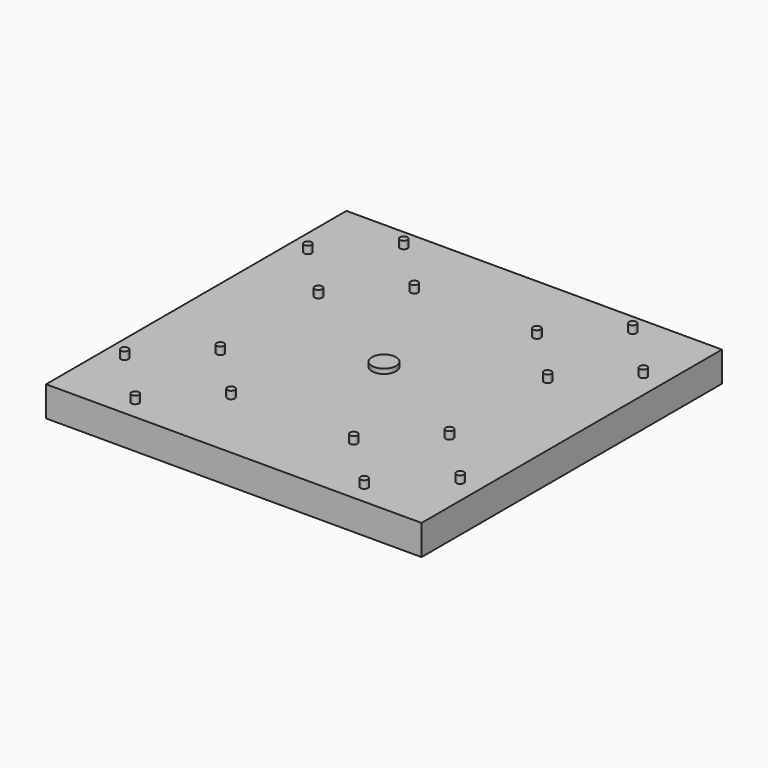
from build123d import *

# Parameters (mm, degrees)
F0_W            = 1995
F0_H            = 1995
F1_DEPTH        = 160
F2_R            = 20
F3_DEPTH        = 40
F3_COPIES_COUNT = 4
F4_R            = 63.875346373
F5_DEPTH        = 25


# Not quite as in the source:
# - a pattern or mirror of a feature is missing from the dataset's text; its kind, count and spacing are read off the source's solid


with BuildPart() as f1:
    # F0 (on Top) → F1 (new body)
    with BuildSketch(Plane.XY):
        Rectangle(F0_W, F0_H)
    extrude(amount=F1_DEPTH)

    # F2 (on face) → F3 (join)
    with BuildSketch(Plane.XY.offset(160)):
        with Locations((-608.5912703474, 891.433982822)):
            Circle(F2_R)
        with Locations((-325.7485578728, 608.5912703474)):
            Circle(F2_R)
        with Locations((-608.5912703474, 325.7485578728)):
            Circle(F2_R)
        with Locations((-891.433982822, 608.5912703474)):
            Circle(F2_R)
    f3 = extrude(amount=F3_DEPTH)

    # F3_copies: F3 ×4 about axis
    f3_copies_axis = Axis((0, 0, 0), (0, 0, 1))
    for i in range(1, F3_COPIES_COUNT):
        add(f3.rotate(f3_copies_axis, i * 360 / F3_COPIES_COUNT))

    # F4 (on face) → F5 (join)
    with BuildSketch(Plane.XY.offset(160)):
        Circle(F4_R)
    extrude(amount=F5_DEPTH)


solid = f1.part
